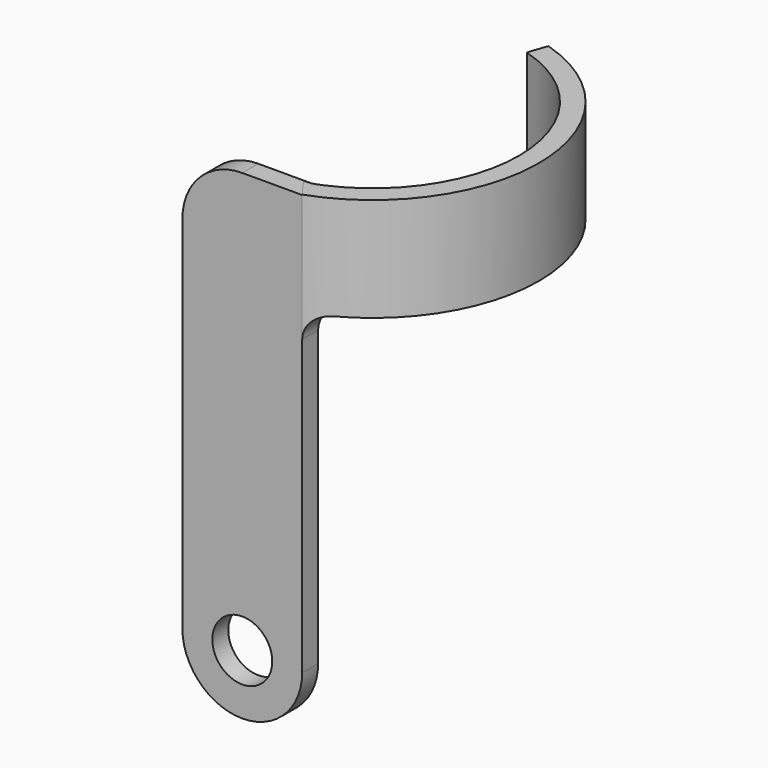
from build123d import *

# Parameters (mm, degrees)
F1_DEPTH = 5
F3_DEPTH = 26
F4_R     = 15
F5_R     = 6


with BuildPart() as f1:
    # F0 (on Front) → F1 (new body)
    with BuildSketch(Plane.XZ):
        with BuildLine():
            Line((15.0000003353, -79.3999582529), (15.0000003353, 25.8973006904))
            Line((15.0000003353, 25.8973006904), (-14.9999996647, 25.8973006904))
            Line((-14.9999996647, 25.8973006904), (-14.9999996647, -79.3999582529))
            ThreePointArc((-14.9999996647, -79.3999582529), (3.353e-07, -64.3999582529), (15.0000003353, -79.3999582529))
        make_face()
        with BuildLine():
            ThreePointArc((-14.9999996647, -79.3999582529), (3.353e-07, -94.3999582529), (15.0000003353, -79.3999582529))
            Line((15.0000003353, -79.3999582529), (7.5000003353, -79.3999582529))
            ThreePointArc((7.5000003353, -79.3999582529), (3.353e-07, -86.8999582529), (-7.4999996647, -79.3999582529))
            Line((-7.4999996647, -79.3999582529), (-14.9999996647, -79.3999582529))
        make_face()
        with BuildLine():
            Line((7.5000003353, -79.3999582529), (15.0000003353, -79.3999582529))
            ThreePointArc((15.0000003353, -79.3999582529), (3.353e-07, -64.3999582529), (-14.9999996647, -79.3999582529))
            Line((-14.9999996647, -79.3999582529), (-7.4999996647, -79.3999582529))
            ThreePointArc((-7.4999996647, -79.3999582529), (3.353e-07, -71.8999582529), (7.5000003353, -79.3999582529))
        make_face()
    extrude(amount=F1_DEPTH)

    # F2 (on Top) → F3 (join)
    with BuildSketch(Plane.XY):
        with BuildLine():
            ThreePointArc((11.6990586319, 69.4567795833), (37.8389339862, 34.4401238089), (11.9304887253, -0.7481090158))
            Line((11.9304887253, -0.7481090158), (14.999749139, -4.999996163))
            ThreePointArc((14.999749139, -4.999996163), (42.8296580573, 35.2079426128), (13.3109600907, 74.1929223018))
            Line((13.3109600907, 74.1929223018), (11.6990586319, 69.4567795833))
        make_face()
    extrude(amount=F3_DEPTH)

    # F4
    f4_edges = [f1.edges().sort_by_distance(p)[0] for p in [
        (-15, -2.5, 25.897301),
    ]]
    fillet(f4_edges, radius=F4_R)

    # F5
    f5_edges = [f1.edges().sort_by_distance(p)[0] for p in [
        (15, -2.499954, 0),
    ]]
    fillet(f5_edges, radius=F5_R)


solid = f1.part
